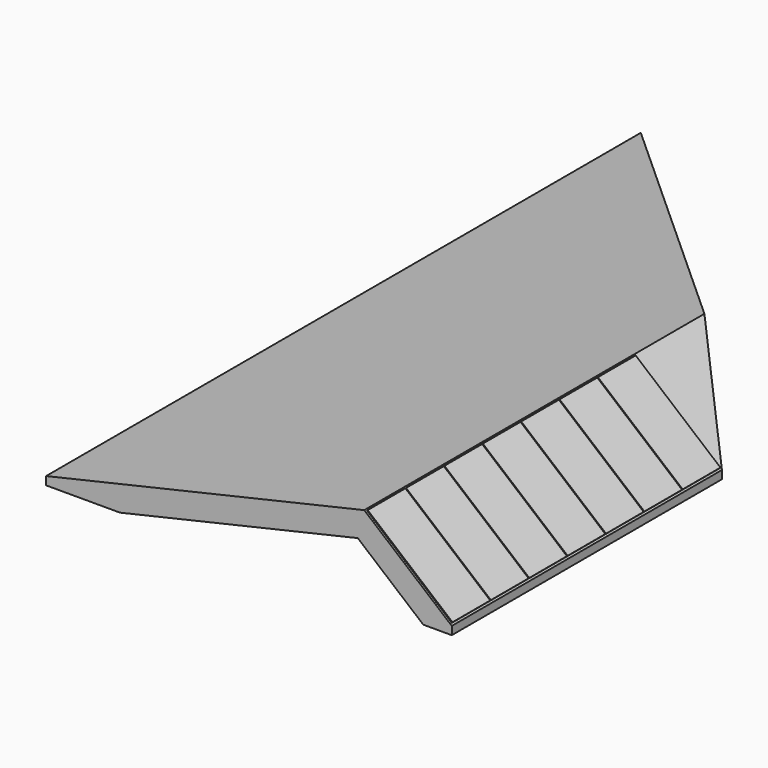
from build123d import *

# Parameters (mm, degrees)
F1_DEPTH = 19000
F3_DEPTH = 1991.7127787042
F4_W     = 2700
F4_H     = 1150
F5_DEPTH = 25


# Not quite as in the source:
# - a feature names something its author has since deleted; it is built from what else it names


with BuildPart() as f1:
    # F0 (on Front) → F1 (new body)
    with BuildSketch(Plane.XZ):
        Polygon((8627.0515179848, 1991.7117787042), (866.2951748568, 200), (866.2951748568, 0), (2667.2468895515, 0), (8470.5403543473, 1339.7958647882), (10067.2468895515, 0), (10762.3304671489, 0), (10762.3304671489, 200), align=None)
    extrude(amount=-F1_DEPTH)

    # F2 (on face) → F3 (cut, through all)
    with BuildSketch(Plane(origin=(0, 0, 0), x_dir=(1, 0, 0), z_dir=(0, 0, -1))):
        Polygon((2667.2468895515, -16332.7531104485), (2667.2468895515, -19000), (11151.2481142848, -19000), (11151.2481142848, -7848.7518857152), align=None)
        Polygon((866.2951748568, -18133.7048251432), (866.2951748568, -19000), (2667.2468895515, -19000), (2667.2468895515, -16332.7531104485), align=None)
    extrude(amount=-F3_DEPTH, mode=Mode.SUBTRACT)

    # F4 (on face) → F5 (join)
    with BuildSketch(Plane(origin=(4545.2164723408, 0, 5416.7780600306), x_dir=(0.7660444431, 0, -0.6427876097), z_dir=(0.6427876097, 0, 0.7660444431))):
        with Locations((6715.8659274322, 625)):
            Rectangle(F4_W, F4_H)
        with Locations((6715.8659274322, 1795)):
            Rectangle(F4_W, F4_H)
        with Locations((6715.8659274322, 2965)):
            Rectangle(F4_W, F4_H)
        with Locations((6715.8659274322, 4135)):
            Rectangle(F4_W, F4_H)
        with Locations((6715.8659274322, 5305)):
            Rectangle(F4_W, F4_H)
        with Locations((6715.8659274322, 6475)):
            Rectangle(F4_W, F4_H)
        with Locations((6715.8659274322, 7645)):
            Rectangle(F4_W, F4_H)
    extrude(amount=F5_DEPTH)


solid = f1.part
